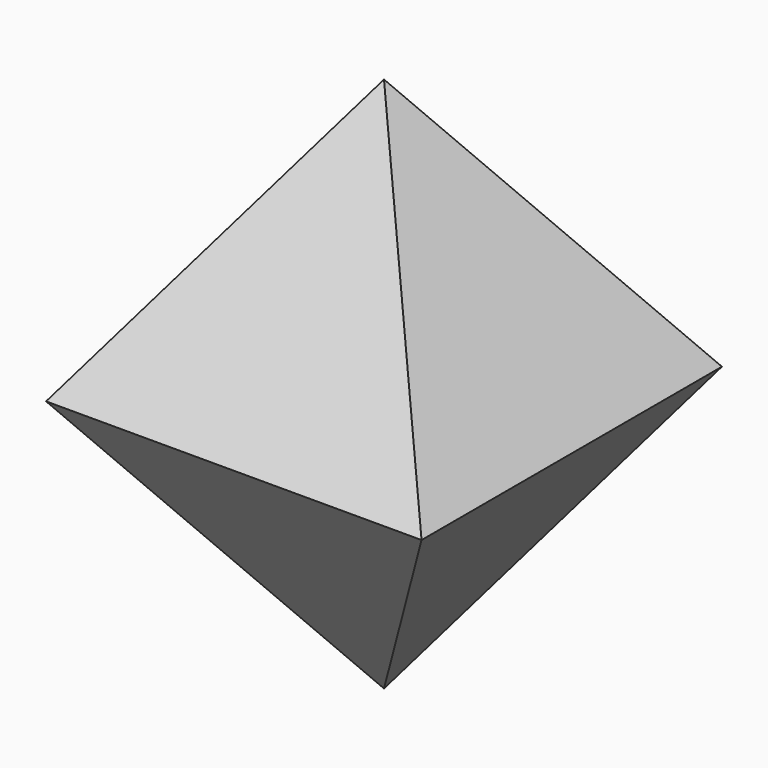
from build123d import *

# Parameters (mm, degrees)
F0_W      = 25.4
F0_H      = 25.4
F1_DEPTH  = 25.4
F1_TAPER  = 35
F1_FACE_W = 25.4
F1_FACE_H = 25.4


# Not quite as in the source:
# - an extrude whose draft closes it to a point is written as a loft to that point


with BuildPart() as f1:
    # F0 (on Top) → F1 (new body)
    with BuildSketch(Plane.XY):
        Rectangle(F0_W, F0_H)
    extrude(amount=F1_DEPTH, taper=F1_TAPER)

    # F1_face (on face) → F2 section 0
    with BuildSketch(Plane(origin=(0, 0, 0), x_dir=(1, 0, 0), z_dir=(0, 0, -1)), mode=Mode.PRIVATE) as f2_s0:
        Rectangle(F1_FACE_W, F1_FACE_H)
    loft([f2_s0.sketch, Vertex(0, 0, -18.1374796856)], ruled=True)


solid = f1.part
